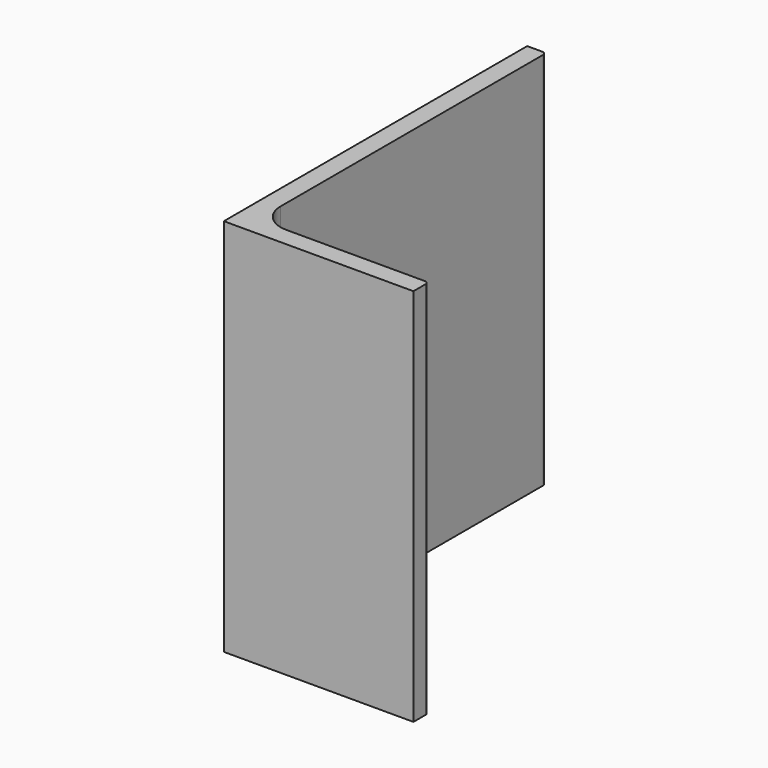
from build123d import *

# Parameters (mm, degrees)
F1_DEPTH = 100
F2_R     = 1


# Not quite as in the source:
# - a feature names something its author has since deleted; it is built from what else it names


with BuildPart() as f1:
    # F0 (on Top) → F1 (new body)
    with BuildSketch(Plane.XY):
        with BuildLine():
            Line((-25, 50), (-25, -50))
            Line((-25, -50), (25, -50))
            Line((25, -50), (25, -45))
            Line((25, -45), (-12.5, -45))
            ThreePointArc((-12.5, -45), (-17.8033008589, -42.8033008589), (-20, -37.5))
            Line((-20, -37.5), (-20, 50))
            Line((-20, 50), (-25, 50))
        make_face()
    extrude(amount=F1_DEPTH)

    # F2
    f2_edges = [f1.edges().sort_by_distance(p)[0] for p in [
        (-20, 50, 50),
        (25, -45, 50),
    ]]
    fillet(f2_edges, radius=F2_R)


solid = f1.part
